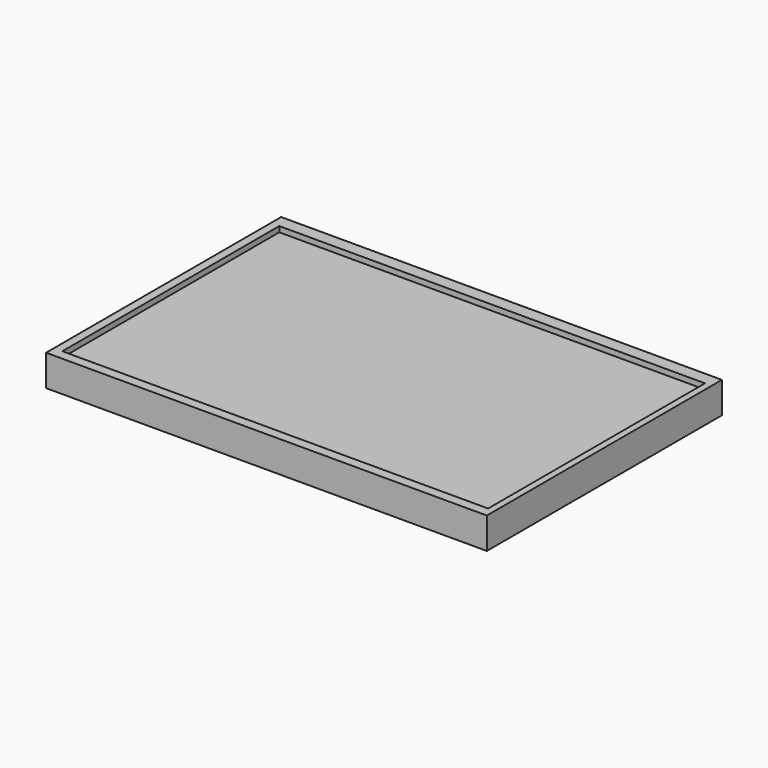
from build123d import *

# Parameters (mm, degrees)
F0_W      = 1200
F0_H      = 800
F1_DEPTH  = 60
F4_DEPTH  = 25
F5_W      = 1136.9413696229
F5_H      = 692.619483918
F6_DEPTH  = 30
F7_W      = 1159.0888965875
F7_H      = 738.1461262703
F8_DEPTH  = 15
F9_W      = 180.6832998991
F9_H      = 355.1081307232
F9_W_2    = 16.8206766248
F9_W_3    = 982.4556671083
F9_H_2    = 21.863527596
F9_H_3    = 568.6533860862
F10_DEPTH = 15


# Not quite as in the source:
# - the program builds the solid bodies; features that only make, move or delete a surface that nothing else refers to are left out


with BuildPart() as f1:
    # F0 (on Top) → F1 (new body)
    with BuildSketch(Plane.XY):
        with Locations((600, 400)):
            Rectangle(F0_W, F0_H)
    extrude(amount=F1_DEPTH)

    # F4 (add): a face of the model
    f4_faces = [f1.faces().sort_by_distance(p)[0] for p in [
        (600, 400, 0),
    ]]
    extrude(f4_faces, amount=F4_DEPTH)

    # F5 (on face) → F6 (cut)
    with BuildSketch(Plane(origin=(0, 0, -25), x_dir=(1, 0, 0), z_dir=(0, 0, -1))):
        with Locations((594.3454820663, -399.9507818371)):
            Rectangle(F5_W, F5_H)
    extrude(amount=-F6_DEPTH, mode=Mode.SUBTRACT)

    # F7 (on face) → F8 (cut)
    with BuildSketch(Plane.XY.offset(60)):
        with Locations((602.350092493, 395.9690630436)):
            Rectangle(F7_W, F7_H)
    extrude(amount=-F8_DEPTH, mode=Mode.SUBTRACT)

    # F9 (on face) → F10 (cut)
    with BuildSketch(Plane(origin=(0, 0, -25), x_dir=(1, 0, 0), z_dir=(0, 0, -1))):
        with Locations((-90.3416499496, -193.3716591448)):
            Rectangle(F9_W, F9_H)
        with Locations((8.4103383124, -193.3716591448)):
            Rectangle(F9_W_2, F9_H)
        with Locations((517.1026308089, -42.7092760801)):
            Rectangle(F9_W_3, F9_H_2)
        Polygon((1162.8161668777, -53.6410398781), (1008.3304643631, -53.6410398781), (1008.3304643631, -622.2944259644), (25.8747972548, -622.2944259644), (25.8747972548, -746.2605237961), (1162.8161668777, -746.2605237961), align=None)
        with Locations((517.1026308089, -337.9677329212)):
            Rectangle(F9_W_3, F9_H_3)
        Polygon((25.8747972548, -15.8175937831), (25.8747972548, -31.7775122821), (1008.3304643631, -31.7775122821), (1008.3304643631, -53.6410398781), (1162.8161668777, -53.6410398781), (1162.8161668777, -746.2605237961), (25.8747972548, -746.2605237961), (25.8747972548, -781.8935513496), (1179.8995733261, -781.8935513496), (1179.8995733261, -15.8175937831), align=None)
    extrude(amount=-F10_DEPTH, mode=Mode.SUBTRACT)


solid = f1.part
